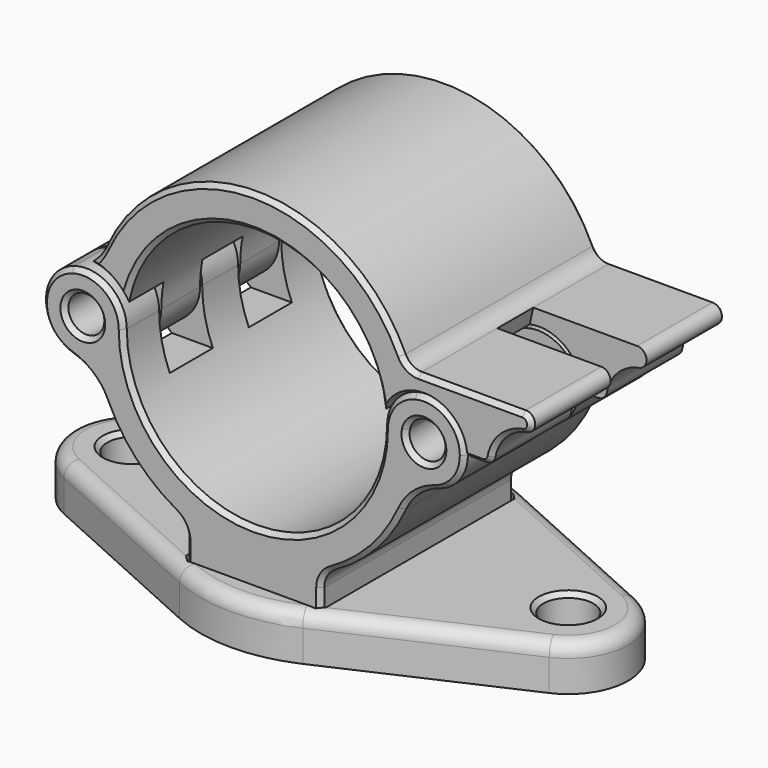
from build123d import *

# Parameters (mm, degrees)
F3_R           = 2.794
F4_DEPTH       = 5
F2_R           = 2
F5_DEPTH       = 13.5
F6_DEPTH       = 13.5
F7_D           = 3.5
F7_CBORE_D     = 6
F7_CBORE_DEPTH = 1.5
F8_D           = 2.3
F8_DEPTH       = 9.5
F8_TIP         = 0.6909897119
F9_W           = 12
F9_H           = 6
F9_H_2         = 4.8
F10_DEPTH      = 14.75
F11_DEPTH      = 8.2
F12_DEPTH      = 2.8
F13_DEPTH      = 2.5
F14_SIZE       = 0.5
F14_2_SIZE     = 0.5
F14_3_SIZE     = 0.5
F15_R          = 1.75
F16_DEPTH      = 1
F17_T1_DEPTH   = 22.1300005366
F17_T3_DEPTH   = 22.1300005366
F17_T5_DEPTH   = 22.1300005366
F17_T7_DEPTH   = 22.1300005366
F17_T10_ANGLE  = 48.6121358442
F17_T12_ANGLE  = 131.3878641558
F17_T14_ANGLE  = 131.3878641558
F17_T16_ANGLE  = 48.6121358442


# Not quite as in the source:
# - a fillet or chamfer that OpenCascade refuses, or shapes differently, is made with other operations: its cross-section is extruded or revolved along the edge and cut away or added


with BuildPart() as f4:
    # F3 (on offset) → F4 (new body)
    with BuildSketch(Plane.XY.offset(-4)):
        with BuildLine():
            Line((-6.8636525628, 15.1970139668), (-27.0320429916, 6.0880650012))
            ThreePointArc((-27.0320429916, 6.0880650012), (-30.9626, 0), (-27.0320429916, -6.0880650012))
            Line((-27.0320429916, -6.0880650012), (-6.8636525628, -15.1970139668))
            ThreePointArc((-6.8636525628, -15.1970139668), (0, -16.6751), (6.8636525628, -15.1970139668))
            Line((6.8636525628, -15.1970139668), (27.0320429916, -6.0880650012))
            ThreePointArc((27.0320429916, -6.0880650012), (30.9626, 0), (27.0320429916, 6.0880650012))
            Line((27.0320429916, 6.0880650012), (6.8636525628, 15.1970139668))
            ThreePointArc((6.8636525628, 15.1970139668), (0, 16.6751), (-6.8636525628, 15.1970139668))
        make_face()
        with Locations((-24.2824, 0)):
            Circle(F3_R, mode=Mode.SUBTRACT)
        with Locations((24.2824, 0)):
            Circle(F3_R, mode=Mode.SUBTRACT)
    extrude(amount=F4_DEPTH)

    # F7 (through all)
    with Locations(Plane(origin=(0, 0, -4), x_dir=(1, 0, 0), z_dir=(0, 0, -1))):
        with Locations((0, -9), (0, 9)):
            CounterBoreHole(F7_D / 2, F7_CBORE_D / 2, F7_CBORE_DEPTH)

    # F14
    f14_edges = [f4.edges().sort_by_distance(p)[0] for p in [
        (21.4884, 0, 1),
        (-27.0764, 0, 1),
        (-3, -9, -4),
        (-3, 9, -4),
    ]]
    chamfer(f14_edges, length=F14_SIZE)

    # F15 (on face) → F16 (cut)
    with BuildSketch(Plane.XY.offset(1)):
        with BuildLine():
            Line((7.5, 13), (7, 13.5))
            Line((7, 13.5), (-7, 13.5))
            Line((-7, 13.5), (-7.5, 13))
            Line((-7.5, 13), (-7.5, 9.4233029003))
            Line((-7.5, 9.4233029003), (-4.8055981695, 10.6402155168))
            ThreePointArc((-4.8055981695, 10.6402155168), (0, 11.6751), (4.8055981695, 10.6402155168))
            Line((4.8055981695, 10.6402155168), (7.5, 9.4233029003))
            Line((7.5, 9.4233029003), (7.5, 13))
        make_face()
        with BuildLine():
            Line((7.5, -9.4233029003), (7.5, 9.4233029003))
            Line((7.5, 9.4233029003), (4.8055981695, 10.6402155168))
            ThreePointArc((4.8055981695, 10.6402155168), (0, 11.6751), (-4.8055981695, 10.6402155168))
            Line((-4.8055981695, 10.6402155168), (-7.5, 9.4233029003))
            Line((-7.5, 9.4233029003), (-7.5, -9.4233029003))
            Line((-7.5, -9.4233029003), (-4.8055981695, -10.6402155168))
            ThreePointArc((-4.8055981695, -10.6402155168), (0, -11.6751), (4.8055981695, -10.6402155168))
            Line((4.8055981695, -10.6402155168), (7.5, -9.4233029003))
        make_face()
        with Locations((0, -9)):
            Circle(F15_R, mode=Mode.SUBTRACT)
        with Locations((0, 9)):
            Circle(F15_R, mode=Mode.SUBTRACT)
        Polygon((7.8, 9.2878094558), (7.5, 9.4233029003), (7.5, -9.4233029003), (7.8, -9.2878094558), align=None)
        with BuildLine():
            Line((7.5, -13), (7.5, -9.4233029003))
            Line((7.5, -9.4233029003), (4.8055981695, -10.6402155168))
            ThreePointArc((4.8055981695, -10.6402155168), (0, -11.6751), (-4.8055981695, -10.6402155168))
            Line((-4.8055981695, -10.6402155168), (-7.5, -9.4233029003))
            Line((-7.5, -9.4233029003), (-7.5, -13))
            Line((-7.5, -13), (-7, -13.5))
            Line((-7, -13.5), (7, -13.5))
            Line((7, -13.5), (7.5, -13))
        make_face()
        Polygon((-7.5, -9.4233029003), (-7.5, 9.4233029003), (-7.8, 9.2878094558), (-7.8, -9.2878094558), align=None)
        Polygon((7.8, -9.2878094558), (7.5, -9.4233029003), (7.5, -13), (7, -13.5), (-7, -13.5), (-7.5, -13), (-7.5, -9.4233029003), (-7.8, -9.2878094558), (-7.8, -13.1242640687), (-7.1242640687, -13.8), (7.1242640687, -13.8), (7.8, -13.1242640687), align=None)
        Polygon((-7, 13.5), (7, 13.5), (7.5, 13), (7.5, 9.4233029003), (7.8, 9.2878094558), (7.8, 13.1242640687), (7.1242640687, 13.8), (-7.1242640687, 13.8), (-7.8, 13.1242640687), (-7.8, 9.2878094558), (-7.5, 9.4233029003), (-7.5, 13), align=None)
    extrude(amount=-F16_DEPTH, mode=Mode.SUBTRACT)

    # F17: fillet of radius 1.5 on 8 edges, made by hand

    # F17_s2 → F17_t1 (cut)
    with BuildSketch(Plane(origin=(-20.1683904289, 9.1089489656, 0), x_dir=(0, 0, 1), z_dir=(0.91135969, -0.4116108787, 0))):
        with BuildLine():
            ThreePointArc((-0.5, 16.6751), (0.5606601718, 16.2357601718), (1, 15.1751))
            Line((1, 15.1751), (1, 16.6751))
            Line((1, 16.6751), (-0.5, 16.6751))
        make_face()
    extrude(amount=F17_T1_DEPTH, mode=Mode.SUBTRACT)

    # F17_s4 → F17_t3 (cut)
    with BuildSketch(Plane(origin=(20.1683904289, -9.1089489656, 0), x_dir=(0, 0, 1), z_dir=(-0.91135969, 0.4116108787, 0))):
        with BuildLine():
            ThreePointArc((-0.5, 16.6751), (0.5606601718, 16.2357601718), (1, 15.1751))
            Line((1, 15.1751), (1, 16.6751))
            Line((1, 16.6751), (-0.5, 16.6751))
        make_face()
    extrude(amount=F17_T3_DEPTH, mode=Mode.SUBTRACT)

    # F17_s6 → F17_t5 (cut)
    with BuildSketch(Plane(origin=(0, 0, 0), x_dir=(0, 0, 1), z_dir=(-0.91135969, -0.4116108787, 0))):
        with BuildLine():
            ThreePointArc((-0.5, 16.6751), (0.5606601718, 16.2357601718), (1, 15.1751))
            Line((1, 15.1751), (1, 16.6751))
            Line((1, 16.6751), (-0.5, 16.6751))
        make_face()
    extrude(amount=F17_T5_DEPTH, mode=Mode.SUBTRACT)

    # F17_s8 → F17_t7 (cut)
    with BuildSketch(Plane(origin=(0, 0, 0), x_dir=(0, 0, 1), z_dir=(0.91135969, 0.4116108787, 0))):
        with BuildLine():
            ThreePointArc((-0.5, 16.6751), (0.5606601718, 16.2357601718), (1, 15.1751))
            Line((1, 15.1751), (1, 16.6751))
            Line((1, 16.6751), (-0.5, 16.6751))
        make_face()
    extrude(amount=F17_T7_DEPTH, mode=Mode.SUBTRACT)

    # F17_s9 → F17_t10 (revolve, cut)
    with BuildSketch(Plane(origin=(0, 0, 0), x_dir=(0, 0, 1), z_dir=(0.91135969, -0.4116108787, 0))):
        with BuildLine():
            ThreePointArc((-0.5, -16.6751), (0.5606601718, -16.2357601718), (1, -15.1751))
            Line((1, -15.1751), (1, -16.6751))
            Line((1, -16.6751), (-0.5, -16.6751))
        make_face()
    revolve(axis=Axis((0, 0, 1), (0, 0, 1)), revolution_arc=F17_T10_ANGLE, mode=Mode.SUBTRACT)

    # F17_s11 → F17_t12 (revolve, cut)
    with BuildSketch(Plane(origin=(20.1683904289, 9.1089489656, 0), x_dir=(0, 0, 1), z_dir=(-0.91135969, -0.4116108787, 0))):
        with BuildLine():
            ThreePointArc((-0.5, -16.6751), (0.5606601718, -16.2357601718), (1, -15.1751))
            Line((1, -15.1751), (1, -16.6751))
            Line((1, -16.6751), (-0.5, -16.6751))
        make_face()
    revolve(axis=Axis((24.2824, 0, 1), (0, 0, 1)), revolution_arc=F17_T12_ANGLE, mode=Mode.SUBTRACT)

    # F17_s13 → F17_t14 (revolve, cut)
    with BuildSketch(Plane(origin=(-20.1683904289, -9.1089489656, 0), x_dir=(0, 0, 1), z_dir=(0.91135969, 0.4116108787, 0))):
        with BuildLine():
            ThreePointArc((-0.5, -16.6751), (0.5606601718, -16.2357601718), (1, -15.1751))
            Line((1, -15.1751), (1, -16.6751))
            Line((1, -16.6751), (-0.5, -16.6751))
        make_face()
    revolve(axis=Axis((-24.2824, 0, 1), (0, 0, 1)), revolution_arc=F17_T14_ANGLE, mode=Mode.SUBTRACT)

    # F17_s15 → F17_t16 (revolve, cut)
    with BuildSketch(Plane(origin=(0, 0, 0), x_dir=(0, 0, 1), z_dir=(-0.91135969, 0.4116108787, 0))):
        with BuildLine():
            ThreePointArc((-0.5, -16.6751), (0.5606601718, -16.2357601718), (1, -15.1751))
            Line((1, -15.1751), (1, -16.6751))
            Line((1, -16.6751), (-0.5, -16.6751))
        make_face()
    revolve(axis=Axis((0, 0, 1), (0, 0, 1)), revolution_arc=F17_T16_ANGLE, mode=Mode.SUBTRACT)


with BuildPart() as f5:
    # F2 (on Front) → F5 (new body, symmetric)
    with BuildSketch(Plane.XZ):
        with BuildLine():
            ThreePointArc((14.5, 21), (0, 6.5), (-14.5, 21))
            ThreePointArc((-14.5, 21), (-16.3240379251, 17.3820963289), (-20.3174342105, 16.6971675491))
            ThreePointArc((-20.3174342105, 16.6971675491), (-18.1153427533, 15.468818933), (-16.6124016549, 13.4441670707))
            ThreePointArc((-16.6124016549, 13.4441670707), (-13.385577703, 8.5948071536), (-8.7951807229, 5.0091496145))
            ThreePointArc((-8.7951807229, 5.0091496145), (-7.848018565, 4.0910120039), (-7.5, 2.8186221644))
            Line((-7.5, 2.8186221644), (-7.5, 0))
            Line((-7.5, 0), (7.5, 0))
            Line((7.5, 0), (7.5, 2.8186221644))
            ThreePointArc((7.5, 2.8186221644), (7.848018565, 4.0910120039), (8.7951807229, 5.0091496145))
            ThreePointArc((8.7951807229, 5.0091496145), (13.385577703, 8.5948071536), (16.6124016549, 13.4441670707))
            ThreePointArc((16.6124016549, 13.4441670707), (18.1153427533, 15.468818933), (20.3174342105, 16.6971675491))
            ThreePointArc((20.3174342105, 16.6971675491), (16.3240379251, 17.3820963289), (14.5, 21))
        make_face()
        with BuildLine():
            ThreePointArc((23.5, 21), (21.7703884478, 24.5461172919), (17.9111342897, 25.3662766134))
            ThreePointArc((17.9111342897, 25.3662766134), (15.4538827081, 23.7703884478), (14.5, 21))
            ThreePointArc((14.5, 21), (16.3240379251, 17.3820963289), (20.3174342105, 16.6971675491))
            ThreePointArc((20.3174342105, 16.6971675491), (22.6179036711, 18.3240379251), (23.5, 21))
        make_face()
        with BuildLine():
            ThreePointArc((21, 21), (18.784262425, 19.0116697209), (17.0465427013, 21.4289575528))
            ThreePointArc((17.0465427013, 21.4289575528), (19.215737575, 22.9883302791), (21, 21))
        make_face(mode=Mode.SUBTRACT)
        with BuildLine():
            ThreePointArc((-20.3174342105, 16.6971675491), (-16.3240379251, 17.3820963289), (-14.5, 21))
            ThreePointArc((-14.5, 21), (-16.3240379251, 24.6179036711), (-20.3174342105, 25.3028324509))
            ThreePointArc((-20.3174342105, 25.3028324509), (-23.5, 21), (-20.3174342105, 16.6971675491))
        make_face()
        with Locations((-19, 21)):
            Circle(F2_R, mode=Mode.SUBTRACT)
    extrude(amount=F5_DEPTH, both=True)

    # F8
    with Locations(Plane(origin=(0, 0, -4), x_dir=(1, 0, 0), z_dir=(0, 0, -1))):
        with Locations((0, 9), (0, -9)):
            Hole(F8_D / 2, depth=F8_DEPTH)
            with Locations((0, 0, -(F8_DEPTH + F8_TIP / 2))):  # 118° drill point
                Cone(0, F8_D / 2, F8_TIP, mode=Mode.SUBTRACT)

    # F9 (on offset) → F10 (cut)
    with BuildSketch(Plane.XY.offset(30)):
        with Locations((-17.5, 5.5)):
            Rectangle(F9_W, F9_H)
        with Locations((-17.5, -5.5)):
            Rectangle(F9_W, F9_H)
        with Locations((17.5, 0)):
            Rectangle(F9_W, F9_H_2)
    extrude(amount=-F10_DEPTH, mode=Mode.SUBTRACT)

    # F14#2
    f14_2_edges = [f5.edges().sort_by_distance(p)[0] for p in [
        (0, -13.5, 6.5),
        (0, 13.5, 6.5),
        (-13.385578, 13.5, 8.594807),
        (-21, 13.5, 21),
        (17, 13.5, 21),
        (-21, -13.5, 21),
        (17, -13.5, 21),
        (18.115343, -13.5, 15.468819),
        (18.115343, 13.5, 15.468819),
        (21.675962, 13.5, 24.617904),
        (-21.675962, 13.5, 24.617904),
        (-18.115343, 13.5, 15.468819),
        (-7.848019, 13.5, 4.091012),
        (-7.5, 13.5, 1.409311),
        (7.5, 13.5, 1.409311),
        (7.848019, 13.5, 4.091012),
        (13.385578, 13.5, 8.594807),
        (-21.675962, -13.5, 24.617904),
        (7.848019, -13.5, 4.091012),
        (7.5, -13.5, 1.409311),
        (-1.15, 9, 0),
        (-1.15, -9, 0),
        (-7.5, -13.5, 1.409311),
        (-7.848019, -13.5, 4.091012),
        (-13.385578, -13.5, 8.594807),
        (-18.115343, -13.5, 15.468819),
        (21.675962, -13.5, 24.617904),
        (13.385578, -13.5, 8.594807),
    ]]
    chamfer(f14_2_edges, length=F14_2_SIZE)


with BuildPart() as f6:
    # F2 (on Front) → F6 (new body, symmetric)
    with BuildSketch(Plane.XZ):
        with BuildLine():
            ThreePointArc((-14.2368421053, 23.7499685216), (0.5926428809, 35.4878837107), (14.4138815789, 22.5779790328))
            ThreePointArc((14.4138815789, 22.5779790328), (15.7868713758, 24.6329470743), (17.9942015869, 25.7445621033))
            Line((17.9942015869, 25.7445621033), (18.3796762757, 27.5))
            ThreePointArc((18.3796762757, 27.5), (17.3024140852, 27.814916568), (16.5643996065, 28.6604938272))
            ThreePointArc((16.5643996065, 28.6604938272), (-0.057571912, 39.2499091909), (-16.6124016549, 28.5558329293))
            ThreePointArc((-16.6124016549, 28.5558329293), (-17.2965161194, 27.4101321912), (-18.2169365732, 26.443970212))
            ThreePointArc((-18.2169365732, 26.443970212), (-15.9170543284, 25.5547168942), (-14.2368421053, 23.7499685216))
        make_face()
        with BuildLine():
            Line((18.3796762757, 27.5), (17.9942015869, 25.7445621033))
            ThreePointArc((17.9942015869, 25.7445621033), (22.053225974, 24.7683300216), (23.85, 21))
            Line((23.85, 21), (25.5916730868, 21))
            ThreePointArc((25.5916730868, 21), (26.2312752359, 21.2312938852), (26.5750052528, 21.8181818182))
            ThreePointArc((26.5750052528, 21.8181818182), (27.8060778992, 24.1699939454), (30.1485660603, 25.4187170362))
            ThreePointArc((30.1485660603, 25.4187170362), (30.9952471709, 26.5496718955), (29.9498743711, 27.5))
            Line((29.9498743711, 27.5), (18.3796762757, 27.5))
        make_face()
    extrude(amount=F6_DEPTH, both=True)

    # F2 (on Front) → F11 (join, symmetric)
    with BuildSketch(Plane.XZ):
        with BuildLine():
            ThreePointArc((-20.3174342105, 16.6971675491), (-16.3240379251, 17.3820963289), (-14.5, 21))
            ThreePointArc((-14.5, 21), (-16.3240379251, 24.6179036711), (-20.3174342105, 25.3028324509))
            ThreePointArc((-20.3174342105, 25.3028324509), (-23.5, 21), (-20.3174342105, 16.6971675491))
        make_face()
        with Locations((-19, 21)):
            Circle(F2_R, mode=Mode.SUBTRACT)
        with BuildLine():
            ThreePointArc((-14.5, 21), (-14.4340605951, 22.3812656286), (-14.2368421053, 23.7499685216))
            ThreePointArc((-14.2368421053, 23.7499685216), (-15.9170543284, 25.5547168942), (-18.2169365732, 26.443970212))
            ThreePointArc((-18.2169365732, 26.443970212), (-19.2097801095, 25.7677351586), (-20.3174342105, 25.3028324509))
            ThreePointArc((-20.3174342105, 25.3028324509), (-16.3240379251, 24.6179036711), (-14.5, 21))
        make_face()
    extrude(amount=F11_DEPTH, both=True)

    # F2 (on Front) → F12 (cut, symmetric)
    with BuildSketch(Plane.XZ):
        with BuildLine():
            ThreePointArc((-20.3174342105, 16.6971675491), (-16.3240379251, 17.3820963289), (-14.5, 21))
            ThreePointArc((-14.5, 21), (-16.3240379251, 24.6179036711), (-20.3174342105, 25.3028324509))
            ThreePointArc((-20.3174342105, 25.3028324509), (-23.5, 21), (-20.3174342105, 16.6971675491))
        make_face()
        with Locations((-19, 21)):
            Circle(F2_R, mode=Mode.SUBTRACT)
        with BuildLine():
            ThreePointArc((-14.5, 21), (-14.4340605951, 22.3812656286), (-14.2368421053, 23.7499685216))
            ThreePointArc((-14.2368421053, 23.7499685216), (-15.9170543284, 25.5547168942), (-18.2169365732, 26.443970212))
            ThreePointArc((-18.2169365732, 26.443970212), (-19.2097801095, 25.7677351586), (-20.3174342105, 25.3028324509))
            ThreePointArc((-20.3174342105, 25.3028324509), (-16.3240379251, 24.6179036711), (-14.5, 21))
        make_face()
    extrude(amount=F12_DEPTH, both=True, mode=Mode.SUBTRACT)

    # F2 (on Front) → F13 (cut, symmetric)
    with BuildSketch(Plane.XZ):
        with BuildLine():
            Line((18.3796762757, 27.5), (17.9942015869, 25.7445621033))
            ThreePointArc((17.9942015869, 25.7445621033), (22.053225974, 24.7683300216), (23.85, 21))
            Line((23.85, 21), (25.5916730868, 21))
            ThreePointArc((25.5916730868, 21), (26.2312752359, 21.2312938852), (26.5750052528, 21.8181818182))
            ThreePointArc((26.5750052528, 21.8181818182), (27.8060778992, 24.1699939454), (30.1485660603, 25.4187170362))
            ThreePointArc((30.1485660603, 25.4187170362), (30.9952471709, 26.5496718955), (29.9498743711, 27.5))
            Line((29.9498743711, 27.5), (18.3796762757, 27.5))
        make_face()
    extrude(amount=F13_DEPTH, both=True, mode=Mode.SUBTRACT)

    # F14#3
    f14_3_edges = [f6.edges().sort_by_distance(p)[0] for p in [
        (-0.057572, -13.5, 39.249909),
        (0.592643, -13.5, 35.487884),
        (-15.917054, -13.5, 25.554717),
        (0.592643, 13.5, 35.487884),
        (-0.057572, 13.5, 39.249909),
        (-17.296516, -13.5, 27.410132),
        (-17.296516, 13.5, 27.410132),
        (24.720837, -13.5, 21),
        (26.231275, -13.5, 21.231294),
        (27.806078, -13.5, 24.169994),
        (30.995247, -13.5, 26.549672),
        (24.164775, -13.5, 27.5),
        (17.302414, -13.5, 27.814917),
        (24.720837, 13.5, 21),
        (26.231275, 13.5, 21.231294),
        (27.806078, 13.5, 24.169994),
        (30.995247, 13.5, 26.549672),
        (24.164775, 13.5, 27.5),
        (17.302414, 13.5, 27.814917),
    ]]
    chamfer(f14_3_edges, length=F14_3_SIZE)


solid = Compound([f4.part, f5.part, f6.part])
